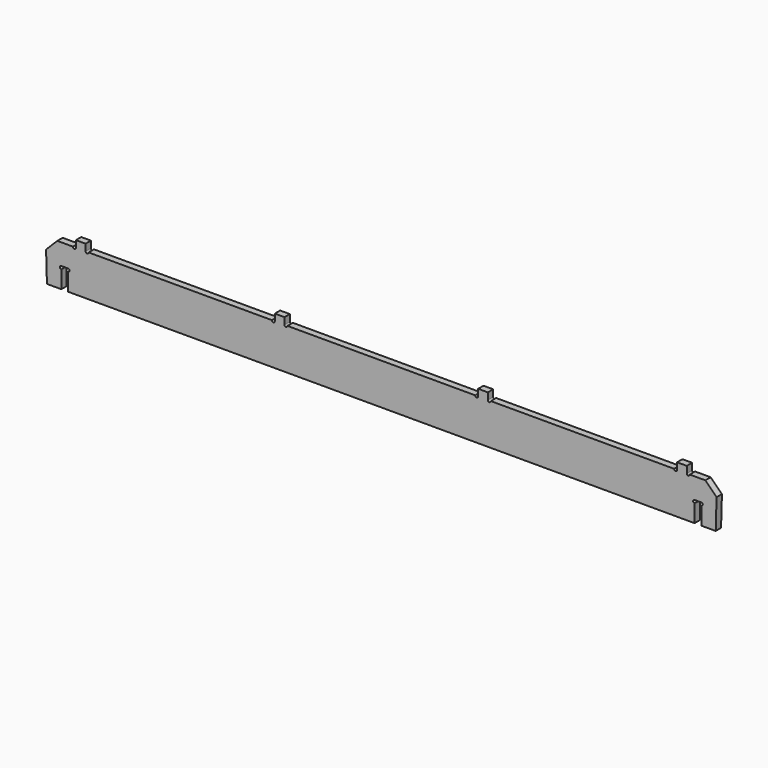
from build123d import *

# Parameters (mm, degrees)
F1_DEPTH = 18


# Not quite as in the source:
# - ends of sketch curves that miss each other by under 0.0002 mm in the source are joined


with BuildPart() as f1:
    # F0 (on Front) → F1 (new body)
    with BuildSketch(Plane.XZ):
        with BuildLine():
            Line((1444.9999982887, 361), (1444.9999982887, 379))
            Line((1444.9999982887, 379), (1418.9999982887, 379))
            Line((1418.9999982887, 379), (1418.9999982887, 361.0032042947))
            Line((1418.9999982887, 361.0032042947), (1418.9999982887, 361))
            ThreePointArc((1418.9999982887, 361), (1414.9978620926, 357.0032048651), (1410.9999984313, 361.0042723931))
            Line((1410.9999984313, 361.0042723931), (918.9999984313, 361.0042723931))
            ThreePointArc((918.9999984313, 361.0042723931), (914.9999984313, 357.0042723931), (910.9999984313, 361.0042723931))
            Line((910.9999984313, 361.0042723931), (910.9999984313, 379.0042723931))
            Line((910.9999984313, 379.0042723931), (884.9999984313, 379.0042723931))
            Line((884.9999984313, 379.0042723931), (884.9999984313, 361.0055952483))
            Line((884.9999984313, 361.0055952483), (884.9999984313, 361.0042723931))
            ThreePointArc((884.9999984313, 361.0042723931), (880.9986755762, 357.005595467), (876.9999986501, 361.0069181034))
            Line((876.9999986501, 361.0069181034), (372.9999978512, 361.1735978616))
            ThreePointArc((372.9999978512, 361.1735978616), (368.9986752099, 357.1749209454), (364.9999982887, 361.1762435819))
            Line((364.9999982887, 361.1762435819), (364.9999982887, 379.1762435819))
            Line((364.9999982887, 379.1762435819), (338.9999982887, 379.1762435819))
            Line((338.9999982887, 379.1762435819), (338.9999982887, 361.1783797782))
            ThreePointArc((338.9999982887, 361.1783797782), (334.9999982887, 357.1783797782), (330.9999982887, 361.1783797782))
            Line((330.9999982887, 361.1783797782), (-161.0000017113, 361.1783797782))
            ThreePointArc((-161.0000017113, 361.1783797782), (-165.0000017113, 357.1783797782), (-169.0000017113, 361.1783797782))
            Line((-169.0000017113, 361.1783797782), (-169.0000017113, 379.1783797782))
            Line((-169.0000017113, 379.1783797782), (-195.0000017113, 379.1783797782))
            Line((-195.0000017113, 379.1783797782), (-195.0000012844, 361.180516095))
            ThreePointArc((-195.0000012844, 361.180516095), (-198.9999999526, 357.1805172846), (-202.9999987156, 361.1805160001))
            Line((-202.9999987156, 361.1805160001), (-215.9862284595, 361.1805160001))
            Line((-215.9862284595, 361.1805160001), (-233.9862284595, 361.1805160001))
            Line((-233.9862284595, 361.1805160001), (-244.90749278, 361.1805160001))
            Line((-244.90749278, 361.1805160001), (-274.9862284595, 331.0746893941))
            Line((-274.9862284595, 331.0746893941), (-272.7034209311, 250.3365797868))
            Line((-272.7034209311, 250.3365797868), (-233.9862284595, 250.3365797868))
            Line((-233.9862284595, 250.3365797868), (-233.9862284595, 297.3365797868))
            ThreePointArc((-233.9862284595, 297.3365797868), (-237.9862284595, 301.3365797868), (-233.9862284595, 305.3365797868))
            Line((-233.9862284595, 305.3365797868), (-215.9862284595, 305.3365797868))
            ThreePointArc((-215.9862284595, 305.3365797868), (-211.9862284595, 301.3365797868), (-215.9862284595, 297.3365797868))
            Line((-215.9862284595, 297.3365797868), (-215.9862284595, 250.3365797868))
            Line((-215.9862284595, 250.3365797868), (-134.9862284595, 250.3365797868))
            Line((-134.9862284595, 250.3365797868), (1385.0137715405, 250.3365797868))
            Line((1385.0137715405, 250.3365797868), (1466.020051896, 250.3365797868))
            Line((1466.020051896, 250.3365797868), (1466.020051896, 297.3365797868))
            ThreePointArc((1466.020051896, 297.3365797868), (1462.020051896, 301.3365797868), (1466.020051896, 305.3365797868))
            Line((1466.020051896, 305.3365797868), (1484.020051896, 305.3365797868))
            ThreePointArc((1484.020051896, 305.3365797868), (1488.020051896, 301.3365797868), (1484.020051896, 297.3365797868))
            Line((1484.020051896, 297.3365797868), (1484.020051896, 250.3365797868))
            Line((1484.020051896, 250.3365797868), (1522.7328349544, 250.3365797868))
            Line((1522.7328349544, 250.3365797868), (1525.0137715405, 331))
            Line((1525.0137715405, 331), (1494.9069982887, 361))
            Line((1494.9069982887, 361), (1466.022162316, 361))
            Line((1466.022162316, 361), (1452.9999982887, 361))
            ThreePointArc((1452.9999982887, 361), (1448.9999982887, 357), (1444.9999982887, 361))
        make_face()
    extrude(amount=F1_DEPTH)


solid = f1.part
